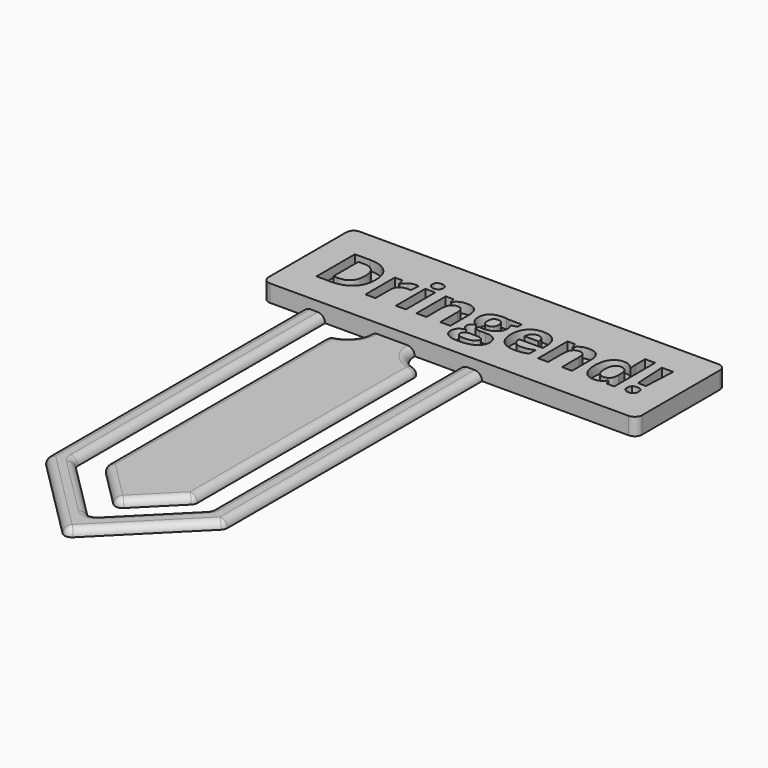
from build123d import *

# Parameters (mm, degrees)
F0_TEXT_SIZE = 8.988190233
F1_DEPTH     = 1
F0_W         = 1.3383977019
F0_H         = 4.9069901053
F2_DEPTH     = 2.3
F3_R         = 0.99999


# Not quite as in the source:
# - a fillet or chamfer is up to 0.001 mm smaller than in the source, because OpenCascade refuses the exact size
# - Text() gives the source's letters only with a copy of the font that has no kerning and outlines rounded to 1/6400 em; it was checked with that copy


with BuildPart() as f1:
    # F0 (on Top) → F1 (new body)
    with BuildSketch(Plane.XY):
        Polygon((20.8785656412, 0), (17.8785656412, 0), (17.8785656412, -43), (29.8785656412, -55), (41.8785656412, -43), (41.8785656412, 0), (38.8785656412, 0), (38.8785656412, -41.7573593129), (29.8785656412, -50.7573593129), (20.8785656412, -41.7573593129), align=None)
        with BuildLine():
            Line((32.8785656412, 0), (26.8785656412, 0))
            ThreePointArc((26.8785656412, 0), (25.9998859847, -2.1213203436), (23.8785656412, -3))
            Line((23.8785656412, -3), (23.8785656412, -40.5147186258))
            Line((23.8785656412, -40.5147186258), (29.8785656412, -46.5147186258))
            Line((29.8785656412, -46.5147186258), (35.8785656412, -40.5147186258))
            Line((35.8785656412, -40.5147186258), (35.8785656412, -3))
            ThreePointArc((35.8785656412, -3), (33.7572452976, -2.1213203436), (32.8785656412, 0))
        make_face()
        with Locations((15.5026199967, 4.2642515161)):
            Text('Dringend!', F0_TEXT_SIZE, font='Open Sans', font_style=FontStyle.BOLD, text_align=(TextAlign.LEFT, TextAlign.BOTTOM))
    extrude(amount=F1_DEPTH)

    # F0 (on Top) → F2 (join)
    with BuildSketch(Plane.XY):
        Polygon((12.5026199967, 0), (17.8785656412, 0), (20.8785656412, 0), (26.8785656412, 0), (32.8785656412, 0), (38.8785656412, 0), (41.8785656412, 0), (62.5026199967, 0), (62.5026199967, 15), (12.5026199967, 15), align=None)
        with BuildLine():
            add(Edge.make_bspline(
                [(20.7649244971, 9.8516757102), (21.6342510212, 9.0223747207), (21.6342510212, 7.5337057134)],
                knots=[0, 0, 0, 1, 1, 1], degree=2))
            add(Edge.make_bspline(
                [(21.6342510212, 7.5337057134), (21.6342510212, 5.9495371848), (20.7319209861, 5.1068943505)],
                knots=[0, 0, 0, 1, 1, 1], degree=2))
            add(Edge.make_bspline(
                [(20.7319209861, 5.1068943505), (19.829590951, 4.2642515161), (18.1274524256, 4.2642515161)],
                knots=[0, 0, 0, 1, 1, 1], degree=2))
            Line((18.1274524256, 4.2642515161), (16.3101527129, 4.2642515161))
            Line((16.3101527129, 4.2642515161), (16.3101527129, 10.6809766996))
            Line((16.3101527129, 10.6809766996), (18.324069087, 10.6809766996))
            add(Edge.make_bspline(
                [(18.324069087, 10.6809766996), (19.895597973, 10.6809766996), (20.7649244971, 9.8516757102)],
                knots=[0, 0, 0, 1, 1, 1], degree=2))
        make_face(mode=Mode.SUBTRACT)
        with BuildLine():
            add(Edge.make_bspline(
                [(24.7527317107, 9.0104372806), (25.1410496168, 9.2625279285), (25.5974811521, 9.2625279285)],
                knots=[0, 0, 0, 1, 1, 1], degree=2))
            add(Edge.make_bspline(
                [(25.5974811521, 9.2625279285), (25.8699356685, 9.2625279285), (26.0496994732, 9.2232045962)],
                knots=[0, 0, 0, 1, 1, 1], degree=2))
            Line((26.0496994732, 9.2232045962), (25.9485823331, 7.9690711778))
            add(Edge.make_bspline(
                [(25.9485823331, 7.9690711778), (25.7856713851, 8.0126077242), (25.5539446057, 8.0126077242)],
                knots=[0, 0, 0, 1, 1, 1], degree=2))
            add(Edge.make_bspline(
                [(25.5539446057, 8.0126077242), (24.9135360516, 8.0126077242), (24.555412847, 7.6832748165)],
                knots=[0, 0, 0, 1, 1, 1], degree=2))
            add(Edge.make_bspline(
                [(24.555412847, 7.6832748165), (24.1972896424, 7.3539419087), (24.1972896424, 6.7612831152)],
                knots=[0, 0, 0, 1, 1, 1], degree=2))
            Line((24.1972896424, 6.7612831152), (24.1972896424, 4.2642515161))
            Line((24.1972896424, 4.2642515161), (22.8588919405, 4.2642515161))
            Line((22.8588919405, 4.2642515161), (22.8588919405, 9.1712416214))
            Line((22.8588919405, 9.1712416214), (23.8728721512, 9.1712416214))
            Line((23.8728721512, 9.1712416214), (24.0708932172, 8.3454516438))
            Line((24.0708932172, 8.3454516438), (24.1354958345, 8.3454516438))
            add(Edge.make_bspline(
                [(24.1354958345, 8.3454516438), (24.3644138045, 8.7583466326), (24.7527317107, 9.0104372806)],
                knots=[0, 0, 0, 1, 1, 1], degree=2))
        make_face(mode=Mode.SUBTRACT)
        with BuildLine():
            Line((38.1486461697, 9.1712416214), (39.8606155281, 9.1712416214))
            Line((39.8606155281, 9.1712416214), (39.8606155281, 8.4901053304))
            Line((39.8606155281, 8.4901053304), (39.0924061441, 8.293488669))
            add(Edge.make_bspline(
                [(39.0924061441, 8.293488669), (39.3030668527, 7.9634535589), (39.3030668527, 7.556176189)],
                knots=[0, 0, 0, 1, 1, 1], degree=2))
            add(Edge.make_bspline(
                [(39.3030668527, 7.556176189), (39.3030668527, 6.7654963294), (38.7518379986, 6.3245132461)],
                knots=[0, 0, 0, 1, 1, 1], degree=2))
            add(Edge.make_bspline(
                [(38.7518379986, 6.3245132461), (38.2006091444, 5.8835301628), (37.2231434566, 5.8835301628)],
                knots=[0, 0, 0, 1, 1, 1], degree=2))
            Line((37.2231434566, 5.8835301628), (36.9815858441, 5.89757421))
            Line((36.9815858441, 5.89757421), (36.783564778, 5.9186402809))
            add(Edge.make_bspline(
                [(36.783564778, 5.9186402809), (36.5771172836, 5.7613469518), (36.5771172836, 5.5675390999)],
                knots=[0, 0, 0, 1, 1, 1], degree=2))
            add(Edge.make_bspline(
                [(36.5771172836, 5.5675390999), (36.5771172836, 5.2782317268), (37.3144297637, 5.2782317268)],
                knots=[0, 0, 0, 1, 1, 1], degree=2))
            Line((37.3144297637, 5.2782317268), (38.1486461697, 5.2782317268))
            add(Edge.make_bspline(
                [(38.1486461697, 5.2782317268), (38.9561788859, 5.2782317268), (39.3796069102, 4.93134376)],
                knots=[0, 0, 0, 1, 1, 1], degree=2))
            add(Edge.make_bspline(
                [(39.3796069102, 4.93134376), (39.8030349344, 4.5844557932), (39.8030349344, 3.9131503351)],
                knots=[0, 0, 0, 1, 1, 1], degree=2))
            add(Edge.make_bspline(
                [(39.8030349344, 3.9131503351), (39.8030349344, 3.0522502394), (39.0853841205, 2.5782636451)],
                knots=[0, 0, 0, 1, 1, 1], degree=2))
            add(Edge.make_bspline(
                [(39.0853841205, 2.5782636451), (38.3677333066, 2.1042770508), (37.0251223905, 2.1042770508)],
                knots=[0, 0, 0, 1, 1, 1], degree=2))
            add(Edge.make_bspline(
                [(37.0251223905, 2.1042770508), (35.9985025374, 2.1042770508), (35.4564023139, 2.4624002553)],
                knots=[0, 0, 0, 1, 1, 1], degree=2))
            add(Edge.make_bspline(
                [(35.4564023139, 2.4624002553), (34.9143020905, 2.8205234599), (34.9143020905, 3.4651452282)],
                knots=[0, 0, 0, 1, 1, 1], degree=2))
            add(Edge.make_bspline(
                [(34.9143020905, 3.4651452282), (34.9143020905, 3.908937121), (35.1909698211, 4.2073731248)],
                knots=[0, 0, 0, 1, 1, 1], degree=2))
            add(Edge.make_bspline(
                [(35.1909698211, 4.2073731248), (35.4676375517, 4.5058091286), (36.0027157515, 4.6336099585)],
                knots=[0, 0, 0, 1, 1, 1], degree=2))
            add(Edge.make_bspline(
                [(36.0027157515, 4.6336099585), (35.7962682571, 4.7206830514), (35.6424859399, 4.9201085222)],
                knots=[0, 0, 0, 1, 1, 1], degree=2))
            add(Edge.make_bspline(
                [(35.6424859399, 4.9201085222), (35.4887036226, 5.119533993), (35.4887036226, 5.3442387488)],
                knots=[0, 0, 0, 1, 1, 1], degree=2))
            add(Edge.make_bspline(
                [(35.4887036226, 5.3442387488), (35.4887036226, 5.6251196936), (35.6509123682, 5.8112033195)],
                knots=[0, 0, 0, 1, 1, 1], degree=2))
            add(Edge.make_bspline(
                [(35.6509123682, 5.8112033195), (35.8131211138, 5.9972869454), (36.1206857483, 6.1784551548)],
                knots=[0, 0, 0, 1, 1, 1], degree=2))
            add(Edge.make_bspline(
                [(36.1206857483, 6.1784551548), (35.7344744493, 6.3441749122), (35.5083652887, 6.7128311523)],
                knots=[0, 0, 0, 1, 1, 1], degree=2))
            add(Edge.make_bspline(
                [(35.5083652887, 6.7128311523), (35.2822561282, 7.0814873923), (35.2822561282, 7.5828598787)],
                knots=[0, 0, 0, 1, 1, 1], degree=2))
            add(Edge.make_bspline(
                [(35.2822561282, 7.5828598787), (35.2822561282, 8.3847749761), (35.8046946855, 8.8236514523)],
                knots=[0, 0, 0, 1, 1, 1], degree=2))
            add(Edge.make_bspline(
                [(35.8046946855, 8.8236514523), (36.3271332428, 9.2625279285), (37.297576907, 9.2625279285)],
                knots=[0, 0, 0, 1, 1, 1], degree=2))
            add(Edge.make_bspline(
                [(37.297576907, 9.2625279285), (37.5040244014, 9.2625279285), (37.7870119533, 9.2253112033)],
                knots=[0, 0, 0, 1, 1, 1], degree=2))
            add(Edge.make_bspline(
                [(37.7870119533, 9.2253112033), (38.0699995051, 9.1880944781), (38.1486461697, 9.1712416214)],
                knots=[0, 0, 0, 1, 1, 1], degree=2))
        make_face(mode=Mode.SUBTRACT)
        with Locations((27.6092909191, 6.7177465688)):
            Rectangle(F0_W, F0_H, mode=Mode.SUBTRACT)
        with BuildLine():
            add(Edge.make_bspline(
                [(27.6113975262, 9.7807532716), (26.8825114745, 9.7807532716), (26.8825114745, 10.4394190871)],
                knots=[0, 0, 0, 1, 1, 1], degree=2))
            add(Edge.make_bspline(
                [(26.8825114745, 10.4394190871), (26.8825114745, 11.0938716885), (27.6113975262, 11.0938716885)],
                knots=[0, 0, 0, 1, 1, 1], degree=2))
            add(Edge.make_bspline(
                [(27.6113975262, 11.0938716885), (28.3402835779, 11.0938716885), (28.3402835779, 10.4394190871)],
                knots=[0, 0, 0, 1, 1, 1], degree=2))
            add(Edge.make_bspline(
                [(28.3402835779, 10.4394190871), (28.3402835779, 10.1276412384), (28.1584131662, 9.954197255)],
                knots=[0, 0, 0, 1, 1, 1], degree=2))
            add(Edge.make_bspline(
                [(28.1584131662, 9.954197255), (27.9765427544, 9.7807532716), (27.6113975262, 9.7807532716)],
                knots=[0, 0, 0, 1, 1, 1], degree=2))
        make_face(mode=Mode.SUBTRACT)
        with BuildLine():
            Line((34.2120997286, 7.4634854772), (34.2120997286, 4.2642515161))
            Line((34.2120997286, 4.2642515161), (32.8737020267, 4.2642515161))
            Line((32.8737020267, 4.2642515161), (32.8737020267, 7.1306415576))
            add(Edge.make_bspline(
                [(32.8737020267, 7.1306415576), (32.8737020267, 7.6615065432), (32.6848095913, 7.9269390361)],
                knots=[0, 0, 0, 1, 1, 1], degree=2))
            add(Edge.make_bspline(
                [(32.6848095913, 7.9269390361), (32.4959171559, 8.1923715289), (32.0830221671, 8.1923715289)],
                knots=[0, 0, 0, 1, 1, 1], degree=2))
            add(Edge.make_bspline(
                [(32.0830221671, 8.1923715289), (31.5212602775, 8.1923715289), (31.2712762367, 7.8173954676)],
                knots=[0, 0, 0, 1, 1, 1], degree=2))
            add(Edge.make_bspline(
                [(31.2712762367, 7.8173954676), (31.0212921958, 7.4424194063), (31.0212921958, 6.5730928822)],
                knots=[0, 0, 0, 1, 1, 1], degree=2))
            Line((31.0212921958, 6.5730928822), (31.0212921958, 4.2642515161))
            Line((31.0212921958, 4.2642515161), (29.682894494, 4.2642515161))
            Line((29.682894494, 4.2642515161), (29.682894494, 9.1712416214))
            Line((29.682894494, 9.1712416214), (30.705301133, 9.1712416214))
            Line((30.705301133, 9.1712416214), (30.8850649376, 8.5434727099))
            Line((30.8850649376, 8.5434727099), (30.959498388, 8.5434727099))
            add(Edge.make_bspline(
                [(30.959498388, 8.5434727099), (31.1842031438, 8.898787105), (31.5767342641, 9.0806575168)],
                knots=[0, 0, 0, 1, 1, 1], degree=2))
            add(Edge.make_bspline(
                [(31.5767342641, 9.0806575168), (31.9692653845, 9.2625279285), (32.4692334662, 9.2625279285)],
                knots=[0, 0, 0, 1, 1, 1], degree=2))
            add(Edge.make_bspline(
                [(32.4692334662, 9.2625279285), (33.3259203478, 9.2625279285), (33.7690100382, 8.799776572)],
                knots=[0, 0, 0, 1, 1, 1], degree=2))
            add(Edge.make_bspline(
                [(33.7690100382, 8.799776572), (34.2120997286, 8.3370252154), (34.2120997286, 7.4634854772)],
                knots=[0, 0, 0, 1, 1, 1], degree=2))
        make_face(mode=Mode.SUBTRACT)
        with BuildLine():
            add(Edge.make_bspline(
                [(43.8631689912, 4.2614427067), (43.4643180497, 4.1757740185), (42.8885121128, 4.1757740185)],
                knots=[0, 0, 0, 1, 1, 1], degree=2))
            add(Edge.make_bspline(
                [(42.8885121128, 4.1757740185), (41.7045989306, 4.1757740185), (41.0375066867, 4.8302266199)],
                knots=[0, 0, 0, 1, 1, 1], degree=2))
            add(Edge.make_bspline(
                [(41.0375066867, 4.8302266199), (40.3704144429, 5.4846792212), (40.3704144429, 6.6826364507)],
                knots=[0, 0, 0, 1, 1, 1], degree=2))
            add(Edge.make_bspline(
                [(40.3704144429, 6.6826364507), (40.3704144429, 7.9157037983), (40.9869481167, 8.5891158634)],
                knots=[0, 0, 0, 1, 1, 1], degree=2))
            add(Edge.make_bspline(
                [(40.9869481167, 8.5891158634), (41.6034817905, 9.2625279285), (42.6918954515, 9.2625279285)],
                knots=[0, 0, 0, 1, 1, 1], degree=2))
            add(Edge.make_bspline(
                [(42.6918954515, 9.2625279285), (43.7311549472, 9.2625279285), (44.3104718958, 8.6705713374)],
                knots=[0, 0, 0, 1, 1, 1], degree=2))
            add(Edge.make_bspline(
                [(44.3104718958, 8.6705713374), (44.8897888444, 8.0786147462), (44.8897888444, 7.0337376317)],
                knots=[0, 0, 0, 1, 1, 1], degree=2))
            Line((44.8897888444, 7.0337376317), (44.8897888444, 6.3834982445))
            Line((44.8897888444, 6.3834982445), (41.7256650015, 6.3834982445))
            add(Edge.make_bspline(
                [(41.7256650015, 6.3834982445), (41.748135477, 5.8133099266), (42.0641265399, 5.4931056495)],
                knots=[0, 0, 0, 1, 1, 1], degree=2))
            add(Edge.make_bspline(
                [(42.0641265399, 5.4931056495), (42.3801176028, 5.1729013725), (42.9503059207, 5.1729013725)],
                knots=[0, 0, 0, 1, 1, 1], degree=2))
            add(Edge.make_bspline(
                [(42.9503059207, 5.1729013725), (43.3940978135, 5.1729013725), (43.7887355409, 5.2648898819)],
                knots=[0, 0, 0, 1, 1, 1], degree=2))
            add(Edge.make_bspline(
                [(43.7887355409, 5.2648898819), (44.1833732683, 5.3568783913), (44.6131211138, 5.5591126716)],
                knots=[0, 0, 0, 1, 1, 1], degree=2))
            Line((44.6131211138, 5.5591126716), (44.6131211138, 4.5226619853))
            add(Edge.make_bspline(
                [(44.6131211138, 4.5226619853), (44.2620199328, 4.3471113948), (43.8631689912, 4.2614427067)],
                knots=[0, 0, 0, 1, 1, 1], degree=2))
        make_face(mode=Mode.SUBTRACT)
        with BuildLine():
            Line((50.50740774, 7.4634854772), (50.50740774, 4.2642515161))
            Line((50.50740774, 4.2642515161), (49.1690100382, 4.2642515161))
            Line((49.1690100382, 4.2642515161), (49.1690100382, 7.1306415576))
            add(Edge.make_bspline(
                [(49.1690100382, 7.1306415576), (49.1690100382, 7.6615065432), (48.9801176028, 7.9269390361)],
                knots=[0, 0, 0, 1, 1, 1], degree=2))
            add(Edge.make_bspline(
                [(48.9801176028, 7.9269390361), (48.7912251674, 8.1923715289), (48.3783301786, 8.1923715289)],
                knots=[0, 0, 0, 1, 1, 1], degree=2))
            add(Edge.make_bspline(
                [(48.3783301786, 8.1923715289), (47.816568289, 8.1923715289), (47.5665842482, 7.8173954676)],
                knots=[0, 0, 0, 1, 1, 1], degree=2))
            add(Edge.make_bspline(
                [(47.5665842482, 7.8173954676), (47.3166002073, 7.4424194063), (47.3166002073, 6.5730928822)],
                knots=[0, 0, 0, 1, 1, 1], degree=2))
            Line((47.3166002073, 6.5730928822), (47.3166002073, 4.2642515161))
            Line((47.3166002073, 4.2642515161), (45.9782025054, 4.2642515161))
            Line((45.9782025054, 4.2642515161), (45.9782025054, 9.1712416214))
            Line((45.9782025054, 9.1712416214), (47.0006091444, 9.1712416214))
            Line((47.0006091444, 9.1712416214), (47.1803729491, 8.5434727099))
            Line((47.1803729491, 8.5434727099), (47.2548063995, 8.5434727099))
            add(Edge.make_bspline(
                [(47.2548063995, 8.5434727099), (47.4795111553, 8.898787105), (47.8720422756, 9.0806575168)],
                knots=[0, 0, 0, 1, 1, 1], degree=2))
            add(Edge.make_bspline(
                [(47.8720422756, 9.0806575168), (48.264573396, 9.2625279285), (48.7645414777, 9.2625279285)],
                knots=[0, 0, 0, 1, 1, 1], degree=2))
            add(Edge.make_bspline(
                [(48.7645414777, 9.2625279285), (49.6212283593, 9.2625279285), (50.0643180497, 8.799776572)],
                knots=[0, 0, 0, 1, 1, 1], degree=2))
            add(Edge.make_bspline(
                [(50.0643180497, 8.799776572), (50.50740774, 8.3370252154), (50.50740774, 7.4634854772)],
                knots=[0, 0, 0, 1, 1, 1], degree=2))
        make_face(mode=Mode.SUBTRACT)
        with BuildLine():
            add(Edge.make_bspline(
                [(57.5863097509, 4.3414937759), (57.384777673, 4.5367060326), (57.384777673, 4.8920204277)],
                knots=[0, 0, 0, 1, 1, 1], degree=2))
            add(Edge.make_bspline(
                [(57.384777673, 4.8920204277), (57.384777673, 5.2599744654), (57.5820965367, 5.4488669007)],
                knots=[0, 0, 0, 1, 1, 1], degree=2))
            add(Edge.make_bspline(
                [(57.5820965367, 5.4488669007), (57.7794154004, 5.6377593361), (58.1572002712, 5.6377593361)],
                knots=[0, 0, 0, 1, 1, 1], degree=2))
            add(Edge.make_bspline(
                [(58.1572002712, 5.6377593361), (58.5209410947, 5.6377593361), (58.7203665655, 5.4446536866)],
                knots=[0, 0, 0, 1, 1, 1], degree=2))
            add(Edge.make_bspline(
                [(58.7203665655, 5.4446536866), (58.9197920362, 5.251548037), (58.9197920362, 4.8920204277)],
                knots=[0, 0, 0, 1, 1, 1], degree=2))
            add(Edge.make_bspline(
                [(58.9197920362, 4.8920204277), (58.9197920362, 4.5451324609), (58.7182599584, 4.3457069901)],
                knots=[0, 0, 0, 1, 1, 1], degree=2))
            add(Edge.make_bspline(
                [(58.7182599584, 4.3457069901), (58.5167278805, 4.1462815193), (58.1572002712, 4.1462815193)],
                knots=[0, 0, 0, 1, 1, 1], degree=2))
            add(Edge.make_bspline(
                [(58.1572002712, 4.1462815193), (57.7878418288, 4.1462815193), (57.5863097509, 4.3414937759)],
                knots=[0, 0, 0, 1, 1, 1], degree=2))
        make_face(mode=Mode.SUBTRACT)
        with BuildLine():
            add(Edge.make_bspline(
                [(54.8301654802, 4.900446856), (54.373733945, 4.1757740185), (53.4384003988, 4.1757740185)],
                knots=[0, 0, 0, 1, 1, 1], degree=2))
            add(Edge.make_bspline(
                [(53.4384003988, 4.1757740185), (52.5746914936, 4.1757740185), (52.0810432332, 4.8477816789)],
                knots=[0, 0, 0, 1, 1, 1], degree=2))
            add(Edge.make_bspline(
                [(52.0810432332, 4.8477816789), (51.5873949727, 5.5197893393), (51.5873949727, 6.7093201404)],
                knots=[0, 0, 0, 1, 1, 1], degree=2))
            add(Edge.make_bspline(
                [(51.5873949727, 6.7093201404), (51.5873949727, 7.9157037983), (52.0894696615, 8.5891158634)],
                knots=[0, 0, 0, 1, 1, 1], degree=2))
            add(Edge.make_bspline(
                [(52.0894696615, 8.5891158634), (52.5915443503, 9.2625279285), (53.4735105169, 9.2625279285)],
                knots=[0, 0, 0, 1, 1, 1], degree=2))
            add(Edge.make_bspline(
                [(53.4735105169, 9.2625279285), (54.4004176347, 9.2625279285), (54.8877460739, 8.5434727099)],
                knots=[0, 0, 0, 1, 1, 1], degree=2))
            Line((54.8877460739, 8.5434727099), (54.9312826204, 8.5434727099))
            add(Edge.make_bspline(
                [(54.9312826204, 8.5434727099), (54.8301654802, 9.0925949569), (54.8301654802, 9.5223428024)],
                knots=[0, 0, 0, 1, 1, 1], degree=2))
            Line((54.8301654802, 9.5223428024), (54.8301654802, 11.0938716885))
            Line((54.8301654802, 11.0938716885), (56.1727763963, 11.0938716885))
            Line((56.1727763963, 11.0938716885), (56.1727763963, 4.2642515161))
            Line((56.1727763963, 4.2642515161), (55.1461565431, 4.2642515161))
            Line((55.1461565431, 4.2642515161), (54.8877460739, 4.900446856))
            Line((54.8877460739, 4.900446856), (54.8301654802, 4.900446856))
        make_face(mode=Mode.SUBTRACT)
        Polygon((58.9197920362, 10.6809766996), (58.6964916851, 6.3933290776), (57.6263352855, 6.3933290776), (57.4016305297, 10.6809766996), align=None, mode=Mode.SUBTRACT)
        with BuildLine():
            add(Edge.make_bspline(
                [(18.2538488508, 5.3877752952), (20.2200154643, 5.3877752952), (20.2200154643, 7.4985955953)],
                knots=[0, 0, 0, 1, 1, 1], degree=2))
            add(Edge.make_bspline(
                [(20.2200154643, 7.4985955953), (20.2200154643, 9.5658793489), (18.3942893232, 9.5658793489)],
                knots=[0, 0, 0, 1, 1, 1], degree=2))
            Line((18.3942893232, 9.5658793489), (17.6710208904, 9.5658793489))
            Line((17.6710208904, 9.5658793489), (17.6710208904, 5.3877752952))
            Line((17.6710208904, 5.3877752952), (18.2538488508, 5.3877752952))
        make_face()
        with BuildLine():
            add(Edge.make_bspline(
                [(37.297576907, 8.4507819981), (36.5602644269, 8.4507819981), (36.5602644269, 7.5646026173)],
                knots=[0, 0, 0, 1, 1, 1], degree=2))
            add(Edge.make_bspline(
                [(36.5602644269, 7.5646026173), (36.5602644269, 7.1657516757), (36.7421348387, 6.9326204915)],
                knots=[0, 0, 0, 1, 1, 1], degree=2))
            add(Edge.make_bspline(
                [(36.7421348387, 6.9326204915), (36.9240052504, 6.6994893074), (37.297576907, 6.6994893074)],
                knots=[0, 0, 0, 1, 1, 1], degree=2))
            add(Edge.make_bspline(
                [(37.297576907, 6.6994893074), (37.673957373, 6.6994893074), (37.8495079635, 6.9326204915)],
                knots=[0, 0, 0, 1, 1, 1], degree=2))
            add(Edge.make_bspline(
                [(37.8495079635, 6.9326204915), (38.025058554, 7.1657516757), (38.025058554, 7.5646026173)],
                knots=[0, 0, 0, 1, 1, 1], degree=2))
            add(Edge.make_bspline(
                [(38.025058554, 7.5646026173), (38.025058554, 8.4507819981), (37.297576907, 8.4507819981)],
                knots=[0, 0, 0, 1, 1, 1], degree=2))
        make_face()
        with BuildLine():
            add(Edge.make_bspline(
                [(36.3208134215, 4.0290137249), (36.0729359877, 3.8555697415), (36.0729359877, 3.5704755825)],
                knots=[0, 0, 0, 1, 1, 1], degree=2))
            add(Edge.make_bspline(
                [(36.0729359877, 3.5704755825), (36.0729359877, 3.2938078519), (36.3383684805, 3.1358123205)],
                knots=[0, 0, 0, 1, 1, 1], degree=2))
            add(Edge.make_bspline(
                [(36.3383684805, 3.1358123205), (36.6038009734, 2.977816789), (37.0827029842, 2.977816789)],
                knots=[0, 0, 0, 1, 1, 1], degree=2))
            add(Edge.make_bspline(
                [(37.0827029842, 2.977816789), (37.8017582029, 2.977816789), (38.2097377752, 3.1758378551)],
                knots=[0, 0, 0, 1, 1, 1], degree=2))
            add(Edge.make_bspline(
                [(38.2097377752, 3.1758378551), (38.6177173474, 3.3738589212), (38.6177173474, 3.7151292691)],
                knots=[0, 0, 0, 1, 1, 1], degree=2))
            add(Edge.make_bspline(
                [(38.6177173474, 3.7151292691), (38.6177173474, 3.9917969997), (38.3768619373, 4.097127354)],
                knots=[0, 0, 0, 1, 1, 1], degree=2))
            add(Edge.make_bspline(
                [(38.3768619373, 4.097127354), (38.1360065271, 4.2024577083), (37.6304208265, 4.2024577083)],
                knots=[0, 0, 0, 1, 1, 1], degree=2))
            Line((37.6304208265, 4.2024577083), (36.9366448929, 4.2024577083))
            add(Edge.make_bspline(
                [(36.9366448929, 4.2024577083), (36.5686908553, 4.2024577083), (36.3208134215, 4.0290137249)],
                knots=[0, 0, 0, 1, 1, 1], degree=2))
        make_face()
        with BuildLine():
            add(Edge.make_bspline(
                [(43.375840552, 8.0406958187), (43.1258565112, 8.3103415257), (42.7003218798, 8.3103415257)],
                knots=[0, 0, 0, 1, 1, 1], degree=2))
            add(Edge.make_bspline(
                [(42.7003218798, 8.3103415257), (42.2747872485, 8.3103415257), (42.033229636, 8.0406958187)],
                knots=[0, 0, 0, 1, 1, 1], degree=2))
            add(Edge.make_bspline(
                [(42.033229636, 8.0406958187), (41.7916720235, 7.7710501117), (41.7565619054, 7.2752952442)],
                knots=[0, 0, 0, 1, 1, 1], degree=2))
            Line((41.7565619054, 7.2752952442), (43.635655426, 7.2752952442))
            add(Edge.make_bspline(
                [(43.635655426, 7.2752952442), (43.6258245929, 7.7710501117), (43.375840552, 8.0406958187)],
                knots=[0, 0, 0, 1, 1, 1], degree=2))
        make_face()
        with BuildLine():
            add(Edge.make_bspline(
                [(53.1926295722, 5.6054580274), (53.442613613, 5.2431216087), (53.9088759813, 5.2431216087)],
                knots=[0, 0, 0, 1, 1, 1], degree=2))
            add(Edge.make_bspline(
                [(53.9088759813, 5.2431216087), (54.4214837056, 5.2431216087), (54.660934711, 5.5415576125)],
                knots=[0, 0, 0, 1, 1, 1], degree=2))
            add(Edge.make_bspline(
                [(54.660934711, 5.5415576125), (54.9003857164, 5.8399936163), (54.922856192, 6.5548356208)],
                knots=[0, 0, 0, 1, 1, 1], degree=2))
            Line((54.922856192, 6.5548356208), (54.922856192, 6.6994893074))
            add(Edge.make_bspline(
                [(54.922856192, 6.6994893074), (54.922856192, 7.4901691669), (54.6791919724, 7.8321417172)],
                knots=[0, 0, 0, 1, 1, 1], degree=2))
            add(Edge.make_bspline(
                [(54.6791919724, 7.8321417172), (54.4355277528, 8.1741142675), (53.8864055058, 8.1741142675)],
                knots=[0, 0, 0, 1, 1, 1], degree=2))
            add(Edge.make_bspline(
                [(53.8864055058, 8.1741142675), (53.4384003988, 8.1741142675), (53.1905229651, 7.794924992)],
                knots=[0, 0, 0, 1, 1, 1], degree=2))
            add(Edge.make_bspline(
                [(53.1905229651, 7.794924992), (52.9426455313, 7.4157357166), (52.9426455313, 6.691062879)],
                knots=[0, 0, 0, 1, 1, 1], degree=2))
            add(Edge.make_bspline(
                [(52.9426455313, 6.691062879), (52.9426455313, 5.9677944462), (53.1926295722, 5.6054580274)],
                knots=[0, 0, 0, 1, 1, 1], degree=2))
        make_face()
    extrude(amount=F2_DEPTH)

    # F3 (radius 1 in the source; OpenCascade refuses exactly that, so slightly less here)
    f3_edges = [f1.edges().sort_by_distance(p)[0] for p in [
        (17.878566, -43, 0.5),
        (29.878566, -55, 0.5),
        (23.878566, -40.514719, 0.5),
        (29.878566, -46.514719, 0.5),
        (41.878566, -43, 0.5),
        (35.878566, -40.514719, 0.5),
        (20.878566, -41.757359, 0.5),
        (29.878566, -50.757359, 0.5),
        (38.878566, -41.757359, 0.5),
        (41.878566, -21.5, 1),
        (35.878566, -49, 1),
        (23.878566, -49, 1),
        (17.878566, -21.5, 1),
        (26.878566, -43.514719, 1),
        (23.878566, -21.757359, 1),
        (32.878566, -43.514719, 1),
        (35.878566, -21.757359, 1),
        (20.878566, -20.87868, 1),
        (12.50262, 0, 1.15),
        (12.50262, 15, 1.15),
        (62.50262, 15, 1.15),
        (62.50262, 0, 1.15),
        (25.999886, -2.12132, 1),
        (33.757245, -2.12132, 1),
        (23.878566, -3, 0.5),
        (35.878566, -3, 0.5),
        (38.878566, -20.87868, 1),
        (34.378566, -46.257359, 1),
        (25.378566, -46.257359, 1),
    ]]
    fillet(f3_edges, radius=F3_R)


solid = f1.part
